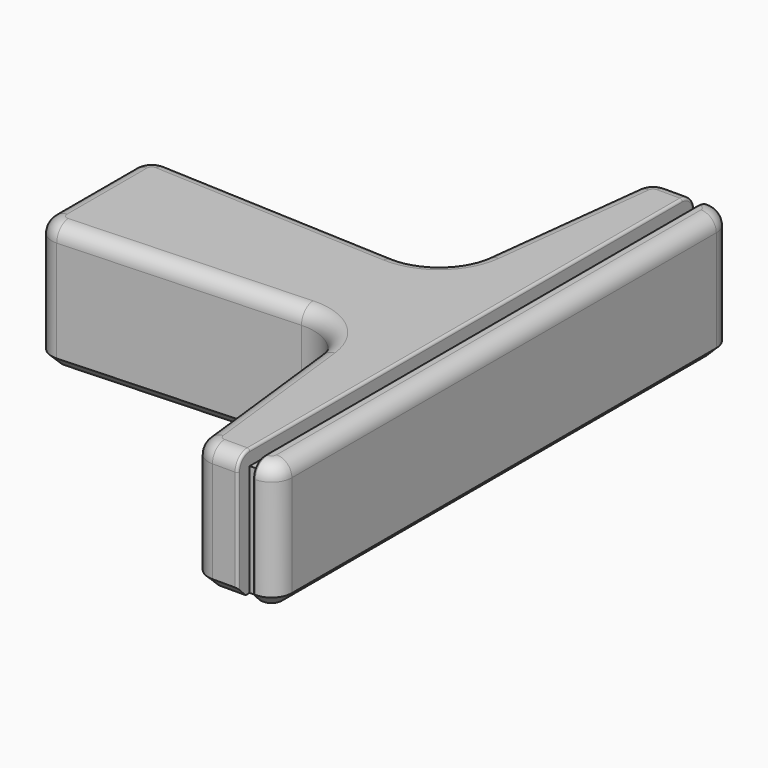
from build123d import *

# Parameters (mm, degrees)
F1_DEPTH = 6.35
F2_R     = 2.54
F3_R     = 1.016
F4_R     = 0.762
F5_SIZE  = 0.508
F6_W     = 0.762
F6_H     = 31.75
F7_DEPTH = 0.762
F8_W     = 0.762
F8_H     = 0.7506295204
F8_H_2   = 0.762
F9_DEPTH = 25.4
F10_R    = 0.12699


# Not quite as in the source:
# - a fillet or chamfer is up to 0.001 mm smaller than in the source, because OpenCascade refuses the exact size


with BuildPart() as f1:
    # F0 (on Top) → F1 (new body)
    with BuildSketch(Plane.XY):
        Polygon((0, -14.2875), (0, 14.2875), (-4.064, 14.2875), (-5.3975, 2.8575), (-20.6375, 3.556), (-20.6375, -3.556), (-5.3975, -2.8575), (-4.064, -14.2875), align=None)
    extrude(amount=F1_DEPTH)

    # F2
    f2_edges = [f1.edges().sort_by_distance(p)[0] for p in [
        (-5.3975, -2.8575, 3.175),
        (-5.3975, 2.8575, 3.175),
    ]]
    fillet(f2_edges, radius=F2_R)

    # F3
    f3_edges = [f1.edges().sort_by_distance(p)[0] for p in [
        (0, 14.2875, 3.175),
        (-4.064, 14.2875, 3.175),
        (0, -14.2875, 3.175),
        (-4.064, -14.2875, 3.175),
        (-20.6375, 3.556, 3.175),
        (-20.6375, -3.556, 3.175),
    ]]
    fillet(f3_edges, radius=F3_R)

    # F4
    f4_edges = [f1.edges().sort_by_distance(p)[0] for p in [
        (-4.645984, 9.299062, 6.35),
        (-3.835156, 14.030405, 6.35),
        (-6.001163, 3.567789, 6.35),
        (-2.087821, 14.2875, 6.35),
        (-13.668668, 3.236595, 6.35),
        (-0.29758, 13.98992, 6.35),
        (-20.323281, 3.22705, 6.35),
        (0, 0, 6.35),
        (-20.6375, 0, 6.35),
        (-0.29758, -13.98992, 6.35),
        (-20.323281, -3.22705, 6.35),
        (-2.087821, -14.2875, 6.35),
        (-13.668668, -3.236595, 6.35),
        (-3.835156, -14.030405, 6.35),
        (-6.001163, -3.567789, 6.35),
        (-4.645984, -9.299062, 6.35),
    ]]
    fillet(f4_edges, radius=F4_R)

    # F5
    f5_edges = [f1.edges().sort_by_distance(p)[0] for p in [
        (-4.645984, 9.299062, 0),
        (-3.835156, 14.030405, 0),
        (-6.001163, 3.567789, 0),
        (-2.087821, 14.2875, 0),
        (-13.668668, 3.236595, 0),
        (-0.29758, 13.98992, 0),
        (-20.323281, 3.22705, 0),
        (0, 0, 0),
        (-20.6375, 0, 0),
        (-0.29758, -13.98992, 0),
        (-20.323281, -3.22705, 0),
        (-2.087821, -14.2875, 0),
        (-13.668668, -3.236595, 0),
        (-3.835156, -14.030405, 0),
        (-6.001163, -3.567789, 0),
        (-4.645984, -9.299062, 0),
    ]]
    chamfer(f5_edges, length=F5_SIZE)

    # F6 (on face) → F7 (cut)
    with BuildSketch(Plane.XY.offset(6.35)):
        with Locations((-1.524, -0.5830885321)):
            Rectangle(F6_W, F6_H)
    extrude(amount=-F7_DEPTH, mode=Mode.SUBTRACT)

    # F8 (on face) → F9 (cut)
    with BuildSketch(Plane.XY.offset(5.588)):
        with Locations((-1.524, 13.9121852398)):
            Rectangle(F8_W, F8_H)
        with Locations((-1.524, -13.9065)):
            Rectangle(F8_W, F8_H_2)
    extrude(amount=-F9_DEPTH, mode=Mode.SUBTRACT)

    # F10 (radius 0.127 in the source; OpenCascade refuses exactly that, so slightly less here)
    f10_edges = [f1.edges().sort_by_distance(p)[0] for p in [
        (-1.143, 0, 6.35),
        (-1.905, 0, 6.35),
    ]]
    fillet(f10_edges, radius=F10_R)


solid = f1.part
